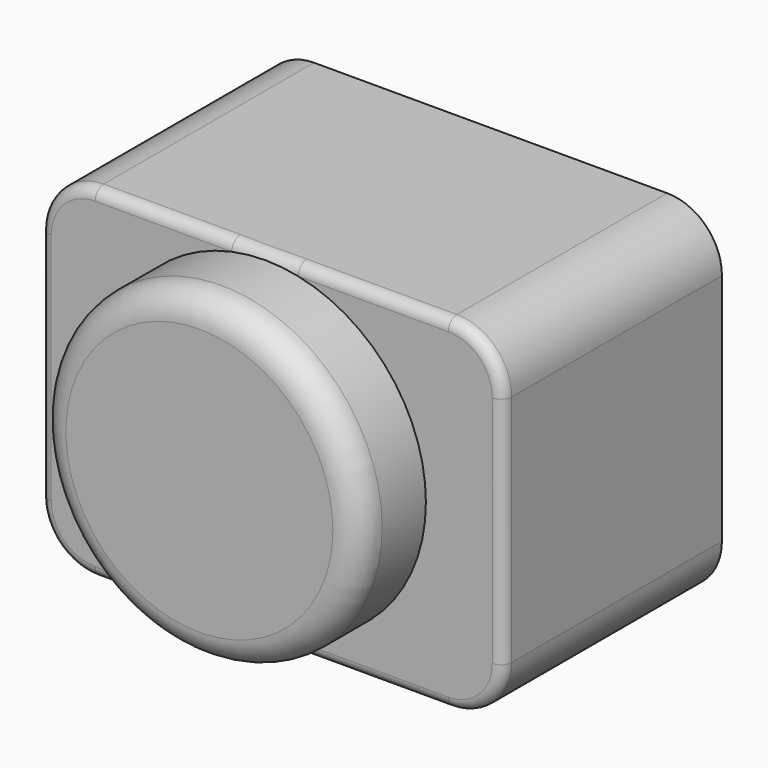
from build123d import *

# Parameters (mm, degrees)
F0_W     = 42.9490916431
F0_H     = 31.8654570729
F1_DEPTH = 25.4
F2_R     = 5.08
F3_T     = -2.54
F4_R     = 14.9347335013
F5_DEPTH = 7.62
F6_R     = 2.54
F7_T     = 2.54
F8_R     = 1


# Not quite as in the source:
# - a shell that OpenCascade refuses in one call is made with other operations: the cavity is built on its own and cut out


with BuildPart() as f1:
    # F0 (on Front) → F1 (new body)
    with BuildSketch(Plane.XZ):
        with Locations((-42.025456205, 33.8281830773)):
            Rectangle(F0_W, F0_H)
    extrude(amount=F1_DEPTH)

    # F2
    f2_edges = [f1.edges().sort_by_distance(p)[0] for p in [
        (-63.500002, -12.7, 49.760912),
        (-20.55091, -12.7, 49.760912),
        (-20.55091, -12.7, 17.895455),
        (-63.500002, -12.7, 17.895455),
    ]]
    fillet(f2_edges, radius=F2_R)

    # F3
    f3_openings = [f1.faces().sort_by_distance(p)[0] for p in [
        (-42.025456, 0, 33.828183),
    ]]
    offset(amount=F3_T, openings=f3_openings)

    # F4 (on face) → F5 (join)
    with BuildSketch(Plane.XZ.offset(25.4)):
        with Locations((-42.6500104368, 34.1481156647)):
            Circle(F4_R)
    extrude(amount=F5_DEPTH)

    # F6
    f6_edges = [f1.edges().sort_by_distance(p)[0] for p in [
        (-57.584744, -33.02, 34.148116),
    ]]
    fillet(f6_edges, radius=F6_R)

    # F7: shell of thickness 2.54, made by hand


with BuildPart() as f7_core1:
    # F7_t2: copy of F1
    add(f1.part)

    # the walls: a layer under each face that stays
    f7_faces = [f7_core1.faces().sort_by_distance(p)[0] for p in [
        (-57.5847439381, -27.94, 34.1481156647),
        (-56.341820086, -25.4, 23.206364053),
        (-42.6500104368, -33.02, 34.1481156647),
        (-42.025456205, -12.7, 49.7609116137),
        (-22.038807935, -12.7, 48.2730140621),
        (-62.012104475, -12.7, 48.2730140621),
        (-20.5509103835, -12.7, 33.8281830773),
        (-63.5000020266, -12.7, 33.8281830773),
        (-22.038807935, -12.7, 19.3833520924),
        (-62.012104475, -12.7, 19.3833520924),
        (-42.025456205, -12.7, 17.8954545408),
        (-60.4322097663, 0, 20.1715586175),
        (-42.025456205, -11.43, 47.2209116137),
        (-23.8348591592, -11.43, 46.4769628379),
        (-23.0909103835, -11.43, 33.8281830773),
        (-23.8348591592, -11.43, 21.1794033166),
        (-42.025456205, -11.43, 20.4354545408),
        (-60.2160532508, -11.43, 21.1794033166),
        (-60.9600020266, -11.43, 33.8281830773),
        (-60.2160532508, -11.43, 46.4769628379),
    ]]
    thicken(f7_faces, amount=-F7_T, mode=Mode.SUBTRACT)

    # F7_s3 → F7_t4 (revolve, cut)
    with BuildSketch(Plane.XY.offset(34.1481156647)):
        Polygon((-27.6898769355, -25.4254), (-30.2552769355, -25.4), (-30.2552769355, -22.86), (-27.7152769355, -22.86), align=None)
    revolve(axis=Axis((-42.6500104368, -25.4, 34.1481156647), (0, -1, 0)), mode=Mode.SUBTRACT)


with BuildPart() as f1_1:
    add(f1.part)

    # what is left inside the walls is the cavity
    f7_cavity = [f7_core1.part.solids().sort_by_distance(p)[0] for p in [
        (-55.019344, -27.94, 34.148116),
    ]]
    add(f7_cavity, mode=Mode.SUBTRACT)

    # F8
    f8_edges = [f1_1.edges().sort_by_distance(p)[0] for p in [
        (-42.025456, -25.4, 49.760912),
        (-22.038808, -25.4, 48.273014),
        (-62.012104, -25.4, 48.273014),
        (-20.55091, -25.4, 33.828183),
        (-63.500002, -25.4, 33.828183),
        (-22.038808, -25.4, 19.383352),
        (-62.012104, -25.4, 19.383352),
        (-42.025456, -25.4, 17.895455),
    ]]
    fillet(f8_edges, radius=F8_R)


solid = f1_1.part
